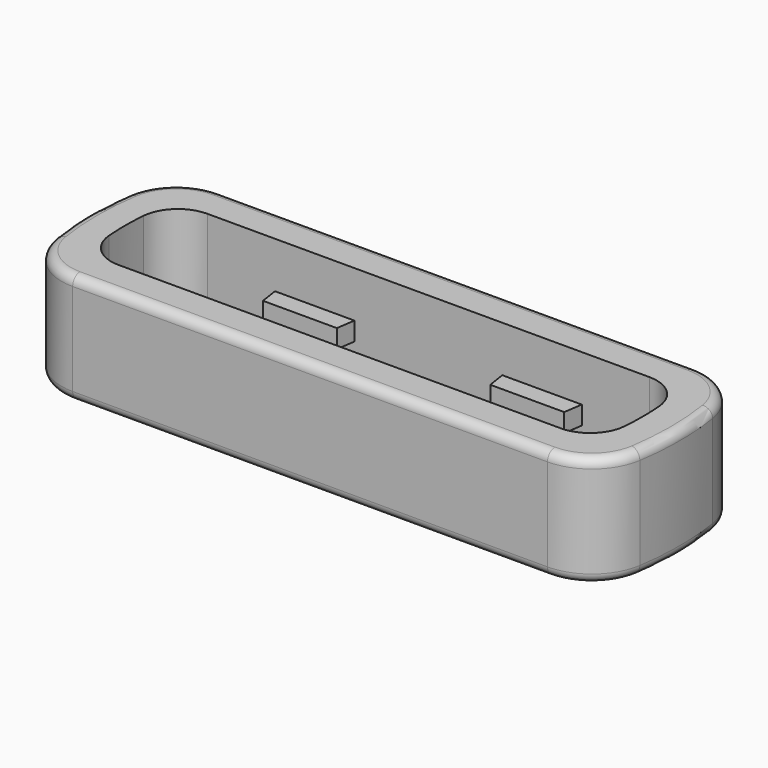
from build123d import *

# Parameters (mm, degrees)
F1_DEPTH = 3
F2_R     = 3
F3_R     = 2
F5_DEPTH = 0.5
F6_R     = 0.5


with BuildPart() as f1:
    # F0 (on Top) → F1 (new body, symmetric)
    with BuildSketch(Plane.XY):
        with BuildLine():
            Line((-15.1986841536, -5), (15.1986841536, -5))
            ThreePointArc((15.1986841536, -5), (16, 0), (15.1986841536, 5))
            Line((15.1986841536, 5), (-15.1986841536, 5))
            ThreePointArc((-15.1986841536, 5), (-16, 0), (-15.1986841536, -5))
        make_face()
        with BuildLine():
            ThreePointArc((13.6747943312, 3), (14, 0), (13.6747943312, -3))
            Line((13.6747943312, -3), (-13.6747943312, -3))
            ThreePointArc((-13.6747943312, -3), (-14, 0), (-13.6747943312, 3))
            Line((-13.6747943312, 3), (13.6747943312, 3))
        make_face(mode=Mode.SUBTRACT)
    extrude(amount=F1_DEPTH, both=True)

    # F2
    f2_edges = [f1.edges().sort_by_distance(p)[0] for p in [
        (-15.198684, 5, 0),
        (15.198684, 5, 0),
        (15.198684, -5, 0),
        (-15.198684, -5, 0),
    ]]
    fillet(f2_edges, radius=F2_R)

    # F3
    f3_edges = [f1.edges().sort_by_distance(p)[0] for p in [
        (13.674794, 3, 0),
        (13.674794, -3, 0),
        (-13.674794, -3, 0),
        (-13.674794, 3, 0),
    ]]
    fillet(f3_edges, radius=F3_R)

    # F4 (on Top) → F5 (join, symmetric)
    with BuildSketch(Plane.XY):
        Polygon((-4, 3), (-8.3, 3), (-8.15, 2), (-4.15, 2), align=None)
        Polygon((8.3, 3), (4, 3), (4.15, 2), (8.15, 2), align=None)
    extrude(amount=F5_DEPTH, both=True)

    # F6
    f6_edges = [f1.edges().sort_by_distance(p)[0] for p in [
        (0, -5, 3),
        (14.796563, -4.278664, 3),
        (16, 0, 3),
        (14.796563, 4.278664, 3),
        (0, 5, 3),
        (-14.796563, -4.278664, 3),
        (-16, 0, 3),
        (-14.796563, 4.278664, 3),
        (-16, 0, -3),
        (-14.796563, 4.278664, -3),
        (-14.796563, -4.278664, -3),
        (0, -5, -3),
        (0, 5, -3),
        (14.796563, -4.278664, -3),
        (16, 0, -3),
        (14.796563, 4.278664, -3),
    ]]
    fillet(f6_edges, radius=F6_R)


solid = f1.part
